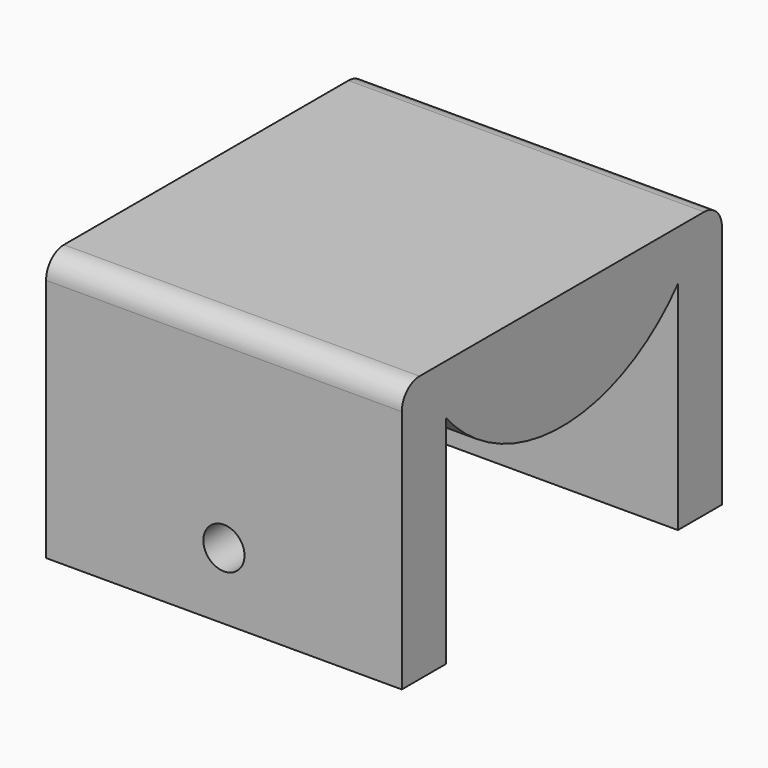
from build123d import *

# Parameters (mm, degrees)
F0_W     = 32
F0_H     = 36
F1_DEPTH = 24
F3_DEPTH = 89
F4_R     = 2
F5_R     = 2
F6_R     = 1.85
F7_DEPTH = 90


# Not quite as in the source:
# - a feature names something its author has since deleted; it is built from what else it names


with BuildPart() as f1:
    # F0 (on Top) → F1 (new body)
    with BuildSketch(Plane.XY):
        Rectangle(F0_W, F0_H)
    extrude(amount=F1_DEPTH)

    # F2 (on face) → F3 (cut)
    with BuildSketch(Plane.YZ.offset(16)):
        with BuildLine():
            ThreePointArc((13.05, 19.5), (0, 13.5), (-13.05, 19.5))
            Line((-13.05, 19.5), (-13.05, 0))
            Line((-13.05, 0), (13.05, 0))
            Line((13.05, 0), (13.05, 19.5))
        make_face()
    extrude(amount=-F3_DEPTH, mode=Mode.SUBTRACT)

    # F4
    f4_edges = [f1.edges().sort_by_distance(p)[0] for p in [
        (0, -18, 24),
    ]]
    fillet(f4_edges, radius=F4_R)

    # F5
    f5_edges = [f1.edges().sort_by_distance(p)[0] for p in [
        (0, 18, 24),
    ]]
    fillet(f5_edges, radius=F5_R)

    # F6 (on face) → F7 (cut)
    with BuildSketch(Plane.XZ.offset(18)):
        with Locations((-24, 6)):
            Circle(F6_R)
        with Locations((0, 6)):
            Circle(F6_R)
        with Locations((24, 6)):
            Circle(F6_R)
    extrude(amount=-F7_DEPTH, mode=Mode.SUBTRACT)


solid = f1.part
